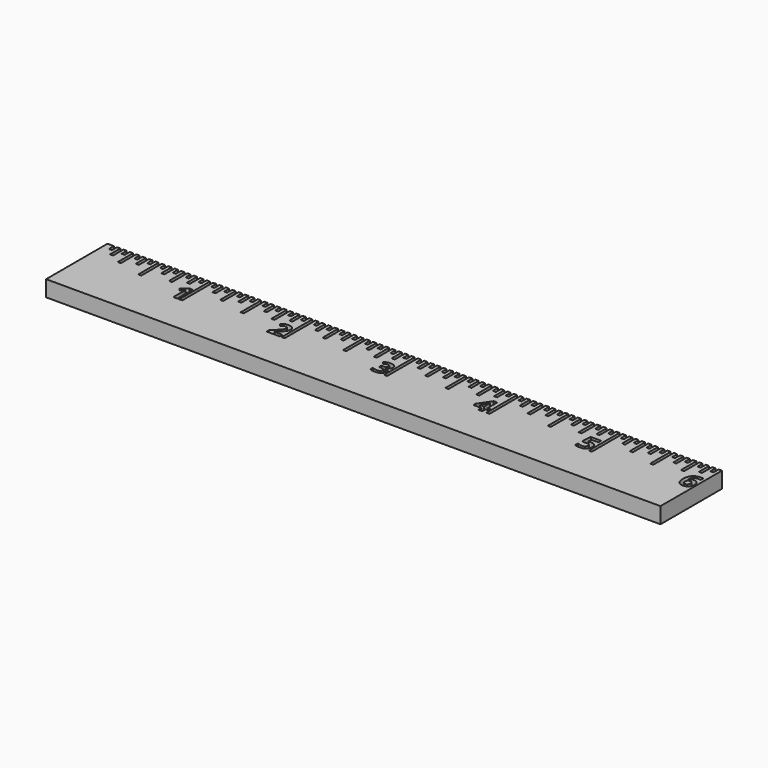
from build123d import *

# Parameters (mm, degrees)
F0_W           = 152.4
F0_H           = 19.05
F1_DEPTH       = 3.175
F3_DEPTH       = 0.79375
F4_TEXT_SIZE   = 6.6972738649
F4_TEXT_SIZE_2 = 6.6224731401
F4_TEXT_SIZE_3 = 6.3550563186
F4_TEXT_SIZE_4 = 6.5505730971
F4_TEXT_SIZE_5 = 6.5812957473
F5_DEPTH       = 1.5875


# Not quite as in the source:
# - Text() gives the source's letters only with a copy of the font that has no kerning and outlines rounded to 1/6400 em; it was checked with that copy


with BuildPart() as f1:
    # F0 (on Top) → F1 (new body)
    with BuildSketch(Plane.XY):
        Rectangle(F0_W, F0_H)
    extrude(amount=F1_DEPTH)

    # F2 (on face) → F3 (join)
    with BuildSketch(Plane.XY.offset(3.175)):
        Polygon((-50.8, 0), (-50.8, 9.525), (-51.6255, 9.525), (-51.6255, 7.9375), (-52.3875, 7.9375), (-52.3875, 9.525), (-53.213, 9.525), (-53.213, 6.35), (-53.975, 6.35), (-53.975, 9.525), (-54.8005, 9.525), (-54.8005, 7.9375), (-55.5625, 7.9375), (-55.5625, 9.525), (-56.388, 9.525), (-56.388, 4.7625), (-57.15, 4.7625), (-57.15, 9.525), (-57.9755, 9.525), (-57.9755, 7.9375), (-58.7375, 7.9375), (-58.7375, 9.525), (-59.563, 9.525), (-59.563, 6.35), (-60.325, 6.35), (-60.325, 9.525), (-61.1505, 9.525), (-61.1505, 7.9375), (-61.9125, 7.9375), (-61.9125, 9.525), (-62.738, 9.525), (-62.738, 3.175), (-63.5, 3.175), (-63.5, 9.525), (-64.3255, 9.525), (-64.3255, 7.9375), (-65.0875, 7.9375), (-65.0875, 9.525), (-65.913, 9.525), (-65.913, 6.35), (-66.675, 6.35), (-66.675, 9.525), (-67.5005, 9.525), (-67.5005, 7.9375), (-68.2625, 7.9375), (-68.2625, 9.525), (-69.088, 9.525), (-69.088, 4.7625), (-69.85, 4.7625), (-69.85, 9.525), (-70.6755, 9.525), (-70.6755, 7.9375), (-71.4375, 7.9375), (-71.4375, 9.525), (-72.263, 9.525), (-72.263, 6.35), (-73.025, 6.35), (-73.025, 9.525), (-73.8505, 9.525), (-73.8505, 7.9375), (-74.6125, 7.9375), (-74.6125, 9.525), (-76.2, 9.525), (-76.2, -9.525), (76.2, -9.525), (76.2, 9.525), (75.3745, 9.525), (75.3745, 7.9375), (74.6125, 7.9375), (74.6125, 9.525), (73.787, 9.525), (73.787, 6.35), (73.025, 6.35), (73.025, 9.525), (72.1995, 9.525), (72.1995, 7.9375), (71.4375, 7.9375), (71.4375, 9.525), (70.612, 9.525), (70.612, 4.7625), (69.85, 4.7625), (69.85, 9.525), (69.0245, 9.525), (69.0245, 7.9375), (68.2625, 7.9375), (68.2625, 9.525), (67.437, 9.525), (67.437, 6.35), (66.675, 6.35), (66.675, 9.525), (65.8495, 9.525), (65.8495, 7.9375), (65.0875, 7.9375), (65.0875, 9.525), (64.262, 9.525), (64.262, 3.175), (63.5, 3.175), (63.5, 9.525), (62.6745, 9.525), (62.6745, 7.9375), (61.9125, 7.9375), (61.9125, 9.525), (61.087, 9.525), (61.087, 6.35), (60.325, 6.35), (60.325, 9.525), (59.4995, 9.525), (59.4995, 7.9375), (58.7375, 7.9375), (58.7375, 9.525), (57.912, 9.525), (57.912, 4.7625), (57.15, 4.7625), (57.15, 9.525), (56.3245, 9.525), (56.3245, 7.9375), (55.5625, 7.9375), (55.5625, 9.525), (54.737, 9.525), (54.737, 6.35), (53.975, 6.35), (53.975, 9.525), (53.1495, 9.525), (53.1495, 7.9375), (52.3875, 7.9375), (52.3875, 9.525), (51.562, 9.525), (51.562, 0), (50.8, 0), (50.8, 9.525), (49.9745, 9.525), (49.9745, 7.9375), (49.2125, 7.9375), (49.2125, 9.525), (48.387, 9.525), (48.387, 6.35), (47.625, 6.35), (47.625, 9.525), (46.7995, 9.525), (46.7995, 7.9375), (46.0375, 7.9375), (46.0375, 9.525), (45.212, 9.525), (45.212, 4.7625), (44.45, 4.7625), (44.45, 9.525), (43.6245, 9.525), (43.6245, 7.9375), (42.8625, 7.9375), (42.8625, 9.525), (42.037, 9.525), (42.037, 6.35), (41.275, 6.35), (41.275, 9.525), (40.4495, 9.525), (40.4495, 7.9375), (39.6875, 7.9375), (39.6875, 9.525), (38.862, 9.525), (38.862, 3.175), (38.1, 3.175), (38.1, 9.525), (37.2745, 9.525), (37.2745, 7.9375), (36.5125, 7.9375), (36.5125, 9.525), (35.687, 9.525), (35.687, 6.35), (34.925, 6.35), (34.925, 9.525), (34.0995, 9.525), (34.0995, 7.9375), (33.3375, 7.9375), (33.3375, 9.525), (32.512, 9.525), (32.512, 4.7625), (31.75, 4.7625), (31.75, 9.525), (30.9245, 9.525), (30.9245, 7.9375), (30.1625, 7.9375), (30.1625, 9.525), (29.337, 9.525), (29.337, 6.35), (28.575, 6.35), (28.575, 9.525), (27.7495, 9.525), (27.7495, 7.9375), (26.9875, 7.9375), (26.9875, 9.525), (26.162, 9.525), (26.162, 0), (25.4, 0), (25.4, 9.525), (24.5745, 9.525), (24.5745, 7.9375), (23.8125, 7.9375), (23.8125, 9.525), (22.987, 9.525), (22.987, 6.35), (22.225, 6.35), (22.225, 9.525), (21.3995, 9.525), (21.3995, 7.9375), (20.6375, 7.9375), (20.6375, 9.525), (19.812, 9.525), (19.812, 4.7625), (19.05, 4.7625), (19.05, 9.525), (18.2245, 9.525), (18.2245, 7.9375), (17.4625, 7.9375), (17.4625, 9.525), (16.637, 9.525), (16.637, 6.35), (15.875, 6.35), (15.875, 9.525), (15.0495, 9.525), (15.0495, 7.9375), (14.2875, 7.9375), (14.2875, 9.525), (13.462, 9.525), (13.462, 3.175), (12.7, 3.175), (12.7, 9.525), (11.8745, 9.525), (11.8745, 7.9375), (11.1125, 7.9375), (11.1125, 9.525), (10.287, 9.525), (10.287, 6.35), (9.525, 6.35), (9.525, 9.525), (8.6995, 9.525), (8.6995, 7.9375), (7.9375, 7.9375), (7.9375, 9.525), (7.112, 9.525), (7.112, 4.7625), (6.35, 4.7625), (6.35, 9.525), (5.5245, 9.525), (5.5245, 7.9375), (4.7625, 7.9375), (4.7625, 9.525), (3.937, 9.525), (3.937, 6.35), (3.175, 6.35), (3.175, 9.525), (2.3495, 9.525), (2.3495, 7.9375), (1.5875, 7.9375), (1.5875, 9.525), (0.762, 9.525), (0.762, 0), (0, 0), (0, 9.525), (-0.8255, 9.525), (-0.8255, 7.9375), (-1.5875, 7.9375), (-1.5875, 9.525), (-2.413, 9.525), (-2.413, 6.35), (-3.175, 6.35), (-3.175, 9.525), (-4.0005, 9.525), (-4.0005, 7.9375), (-4.7625, 7.9375), (-4.7625, 9.525), (-5.588, 9.525), (-5.588, 4.7625), (-6.35, 4.7625), (-6.35, 9.525), (-7.1755, 9.525), (-7.1755, 7.9375), (-7.9375, 7.9375), (-7.9375, 9.525), (-8.763, 9.525), (-8.763, 6.35), (-9.525, 6.35), (-9.525, 9.525), (-10.3505, 9.525), (-10.3505, 7.9375), (-11.1125, 7.9375), (-11.1125, 9.525), (-11.938, 9.525), (-11.938, 3.175), (-12.7, 3.175), (-12.7, 9.525), (-13.5255, 9.525), (-13.5255, 7.9375), (-14.2875, 7.9375), (-14.2875, 9.525), (-15.113, 9.525), (-15.113, 6.35), (-15.875, 6.35), (-15.875, 9.525), (-16.7005, 9.525), (-16.7005, 7.9375), (-17.4625, 7.9375), (-17.4625, 9.525), (-18.288, 9.525), (-18.288, 4.7625), (-19.05, 4.7625), (-19.05, 9.525), (-19.8755, 9.525), (-19.8755, 7.9375), (-20.6375, 7.9375), (-20.6375, 9.525), (-21.463, 9.525), (-21.463, 6.35), (-22.225, 6.35), (-22.225, 9.525), (-23.0505, 9.525), (-23.0505, 7.9375), (-23.8125, 7.9375), (-23.8125, 9.525), (-24.638, 9.525), (-24.638, 0), (-25.4, 0), (-25.4, 9.525), (-26.2255, 9.525), (-26.2255, 7.9375), (-26.9875, 7.9375), (-26.9875, 9.525), (-27.813, 9.525), (-27.813, 6.35), (-28.575, 6.35), (-28.575, 9.525), (-29.4005, 9.525), (-29.4005, 7.9375), (-30.1625, 7.9375), (-30.1625, 9.525), (-30.988, 9.525), (-30.988, 4.7625), (-31.75, 4.7625), (-31.75, 9.525), (-32.5755, 9.525), (-32.5755, 7.9375), (-33.3375, 7.9375), (-33.3375, 9.525), (-34.163, 9.525), (-34.163, 6.35), (-34.925, 6.35), (-34.925, 9.525), (-35.7505, 9.525), (-35.7505, 7.9375), (-36.5125, 7.9375), (-36.5125, 9.525), (-37.338, 9.525), (-37.338, 3.175), (-38.1, 3.175), (-38.1, 9.525), (-38.9255, 9.525), (-38.9255, 7.9375), (-39.6875, 7.9375), (-39.6875, 9.525), (-40.513, 9.525), (-40.513, 6.35), (-41.275, 6.35), (-41.275, 9.525), (-42.1005, 9.525), (-42.1005, 7.9375), (-42.8625, 7.9375), (-42.8625, 9.525), (-43.688, 9.525), (-43.688, 4.7625), (-44.45, 4.7625), (-44.45, 9.525), (-45.2755, 9.525), (-45.2755, 7.9375), (-46.0375, 7.9375), (-46.0375, 9.525), (-46.863, 9.525), (-46.863, 6.35), (-47.625, 6.35), (-47.625, 9.525), (-48.4505, 9.525), (-48.4505, 7.9375), (-49.2125, 7.9375), (-49.2125, 9.525), (-50.038, 9.525), (-50.038, 0), align=None)
    extrude(amount=F3_DEPTH)

    # F4 (on face) → F5 (cut)
    with BuildSketch(Plane.XY.offset(3.96875)):
        with Locations((-54.0243014693, 0)):
            Text('1', F4_TEXT_SIZE, font='Open Sans', font_style=FontStyle.BOLD, text_align=(TextAlign.LEFT, TextAlign.BOTTOM))
        with Locations((-29.3986033648, 0)):
            Text('2', F4_TEXT_SIZE_2, font='Open Sans', font_style=FontStyle.BOLD, text_align=(TextAlign.LEFT, TextAlign.BOTTOM))
        with Locations((-3.7941672177, 0)):
            Text('3', F4_TEXT_SIZE_3, font='Open Sans', font_style=FontStyle.BOLD, text_align=(TextAlign.LEFT, TextAlign.BOTTOM))
        with Locations((21.2949886918, 0)):
            Text('4', F4_TEXT_SIZE_4, font='Open Sans', font_style=FontStyle.BOLD, text_align=(TextAlign.LEFT, TextAlign.BOTTOM))
        with Locations((46.9473078847, 0)):
            Text('5', F4_TEXT_SIZE_5, font='Open Sans', font_style=FontStyle.BOLD, text_align=(TextAlign.LEFT, TextAlign.BOTTOM))
        with Locations((72.2255143651, 0)):
            Text('6', F4_TEXT_SIZE_5, font='Open Sans', font_style=FontStyle.BOLD, text_align=(TextAlign.LEFT, TextAlign.BOTTOM))
    extrude(amount=-F5_DEPTH, mode=Mode.SUBTRACT)


solid = f1.part
